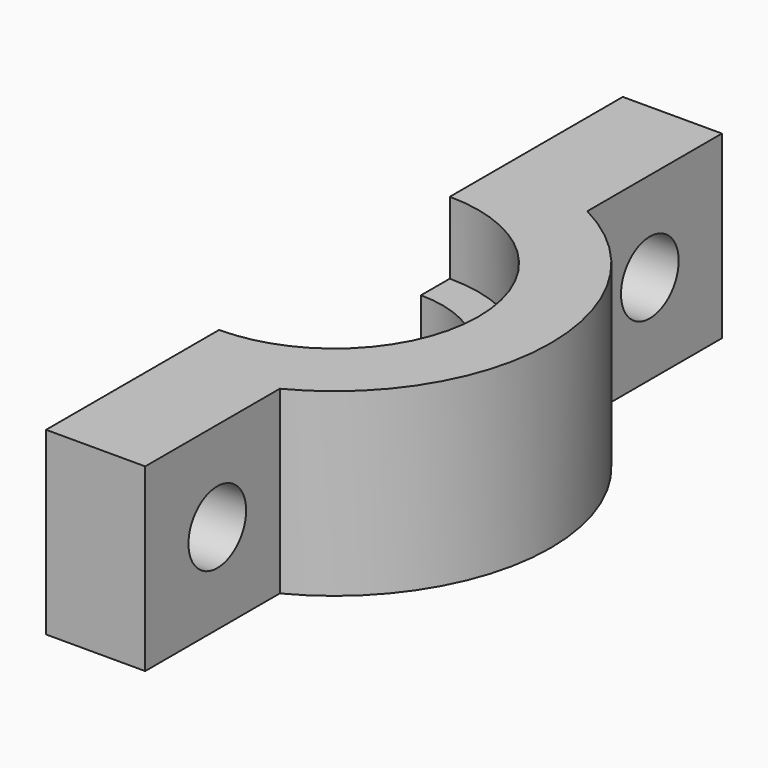
from build123d import *

# Parameters (mm, degrees)
F1_DEPTH = 10
F3_DEPTH = 4
F4_W     = 5.5
F4_H     = 11.188021542
F4_H_2   = 22.7246312633
F4_H_3   = 10.0103956625
F5_DEPTH = 25
F6_DEPTH = 4
F8_D     = 4
F8_DEPTH = 9
F8_TIP   = 1.2017212381


# Not quite as in the source:
# - a feature names something its author has since deleted; it is built from what else it names


with BuildPart() as f1:
    # F0 (on Top) → F1 (new body)
    with BuildSketch(Plane.XY):
        Polygon((60, 11.5470053838), (40, 46.1880215352), (-40, 46.1880215352), (-60, 11.5470053838), (-20, -57.735026919), (20, -57.735026919), align=None)
    extrude(amount=F1_DEPTH)

    # F2 (on face) → F3 (cut)
    with BuildSketch(Plane.XY.offset(10)):
        Polygon((-42.8867513499, 31.188021542), (-48.4529946241, 21.5470053838), (-5.5662432742, -52.7350269258), (5.5662432742, -52.7350269258), (48.4529946241, 21.5470053838), (42.8867513499, 31.188021542), align=None)
    extrude(amount=-F3_DEPTH, mode=Mode.SUBTRACT)

    # F4 (on face) + F1_face (on face) → F5 (cut)
    with BuildSketch(Plane.XY.offset(6)):
        with BuildLine():
            ThreePointArc((-5.5, -10.6653645039), (-12, 0), (-5.5, 10.6653645039))
            Line((-5.5, 10.6653645039), (-5.5, 20))
            Line((-5.5, 20), (-5.5, 31.188021542))
            Line((-5.5, 31.188021542), (-42.8867513499, 31.188021542))
            Line((-42.8867513499, 31.188021542), (-48.4529946241, 21.5470053838))
            Line((-48.4529946241, 21.5470053838), (-11.3457479046, -42.7246312633))
            Line((-11.3457479046, -42.7246312633), (-5.5, -42.7246312633))
            Line((-5.5, -42.7246312633), (-5.5, -20))
            Line((-5.5, -20), (-5.5, -10.6653645039))
        make_face()
        with Locations((2.75, 25.594010771)):
            Rectangle(F4_W, F4_H)
        with Locations((-2.75, 25.594010771)):
            Rectangle(F4_W, F4_H)
        with BuildLine():
            ThreePointArc((-5.5, 10.6653645039), (-2.8298079399, 11.6615688063), (0, 12))
            Line((0, 12), (0, 20))
            Line((0, 20), (-5.5, 20))
            Line((-5.5, 20), (-5.5, 10.6653645039))
        make_face()
        with BuildLine():
            ThreePointArc((-5.5, 5.8094750193), (-2.9600844452, 7.4322204002), (0, 8))
            Line((0, 8), (0, 12))
            ThreePointArc((0, 12), (-2.8298079399, 11.6615688063), (-5.5, 10.6653645039))
            Line((-5.5, 10.6653645039), (-5.5, 5.8094750193))
        make_face()
        with BuildLine():
            ThreePointArc((-5.5, 2.3979157617), (-3.2872865277, 5.0193373352), (0, 6))
            Line((0, 6), (0, 8))
            ThreePointArc((0, 8), (-2.9600844452, 7.4322204002), (-5.5, 5.8094750193))
            Line((-5.5, 5.8094750193), (-5.5, 2.3979157617))
        make_face()
        with BuildLine():
            Line((5.5, -2.3979157617), (5.5, 2.3979157617))
            ThreePointArc((5.5, 2.3979157617), (3.2872865277, 5.0193373352), (0, 6))
            ThreePointArc((0, 6), (-3.2872865277, 5.0193373352), (-5.5, 2.3979157617))
            Line((-5.5, 2.3979157617), (-5.5, -2.3979157617))
            ThreePointArc((-5.5, -2.3979157617), (-3.2872865277, -5.0193373352), (0, -6))
            ThreePointArc((0, -6), (3.2872865277, -5.0193373352), (5.5, -2.3979157617))
        make_face()
        with BuildLine():
            ThreePointArc((-5.5, -2.3979157617), (-6, 0), (-5.5, 2.3979157617))
            Line((-5.5, 2.3979157617), (-5.5, 5.8094750193))
            ThreePointArc((-5.5, 5.8094750193), (-8, 0), (-5.5, -5.8094750193))
            Line((-5.5, -5.8094750193), (-5.5, -2.3979157617))
        make_face()
        with BuildLine():
            ThreePointArc((-5.5, -5.8094750193), (-8, 0), (-5.5, 5.8094750193))
            Line((-5.5, 5.8094750193), (-5.5, 10.6653645039))
            ThreePointArc((-5.5, 10.6653645039), (-12, 0), (-5.5, -10.6653645039))
            Line((-5.5, -10.6653645039), (-5.5, -5.8094750193))
        make_face()
        with BuildLine():
            Line((-5.5, -2.3979157617), (-5.5, 2.3979157617))
            ThreePointArc((-5.5, 2.3979157617), (-6, 0), (-5.5, -2.3979157617))
        make_face()
        with BuildLine():
            Line((0, -8), (0, -6))
            ThreePointArc((0, -6), (-3.2872865277, -5.0193373352), (-5.5, -2.3979157617))
            Line((-5.5, -2.3979157617), (-5.5, -5.8094750193))
            ThreePointArc((-5.5, -5.8094750193), (-2.9600844452, -7.4322204002), (0, -8))
        make_face()
        with BuildLine():
            Line((0, -12), (0, -8))
            ThreePointArc((0, -8), (-2.9600844452, -7.4322204002), (-5.5, -5.8094750193))
            Line((-5.5, -5.8094750193), (-5.5, -10.6653645039))
            ThreePointArc((-5.5, -10.6653645039), (-2.8298079399, -11.6615688063), (0, -12))
        make_face()
        with BuildLine():
            Line((0, -20), (0, -12))
            ThreePointArc((0, -12), (-2.8298079399, -11.6615688063), (-5.5, -10.6653645039))
            Line((-5.5, -10.6653645039), (-5.5, -20))
            Line((-5.5, -20), (0, -20))
        make_face()
        with Locations((-2.75, -31.3623156317)):
            Rectangle(F4_W, F4_H_2)
        with Locations((2.75, -31.3623156317)):
            Rectangle(F4_W, F4_H_2)
        with BuildLine():
            Line((5.5, 20), (5.5, 10.6653645039))
            ThreePointArc((5.5, 10.6653645039), (10.246950766, 6.2449979984), (12, 0))
            ThreePointArc((12, 0), (10.246950766, -6.2449979984), (5.5, -10.6653645039))
            Line((5.5, -10.6653645039), (5.5, -20))
            Line((5.5, -20), (5.5, -42.7246312633))
            Line((5.5, -42.7246312633), (11.3457479046, -42.7246312633))
            Line((11.3457479046, -42.7246312633), (48.4529946241, 21.5470053838))
            Line((48.4529946241, 21.5470053838), (42.8867513499, 31.188021542))
            Line((42.8867513499, 31.188021542), (5.5, 31.188021542))
            Line((5.5, 31.188021542), (5.5, 20))
        make_face()
        Polygon((11.3457479046, -42.7246312633), (5.5, -42.7246312633), (5.5, -52.7350269258), (5.5662432742, -52.7350269258), align=None)
        with Locations((2.75, -47.7298290946)):
            Rectangle(F4_W, F4_H_3)
        with Locations((-2.75, -47.7298290946)):
            Rectangle(F4_W, F4_H_3)
        Polygon((-5.5, -52.7350269258), (-5.5, -42.7246312633), (-11.3457479046, -42.7246312633), (-5.5662432742, -52.7350269258), align=None)
        with BuildLine():
            ThreePointArc((5.5, -2.3979157617), (5.8736700622, -1.2247448714), (6, 0))
            ThreePointArc((6, 0), (5.8736700622, 1.2247448714), (5.5, 2.3979157617))
            Line((5.5, 2.3979157617), (5.5, -2.3979157617))
        make_face()
    with BuildSketch(Plane.XY.offset(10)):
        Polygon((60, 11.5470053838), (40, 46.1880215352), (-40, 46.1880215352), (-60, 11.5470053838), (-20, -57.735026919), (20, -57.735026919), align=None)
        Polygon((-48.4529946241, 21.5470053838), (-42.8867513499, 31.188021542), (42.8867513499, 31.188021542), (48.4529946241, 21.5470053838), (5.5662432742, -52.7350269258), (-5.5662432742, -52.7350269258), align=None, mode=Mode.SUBTRACT)
    extrude(amount=-F5_DEPTH, mode=Mode.SUBTRACT)

    # F4 (on face) → F6 (join)
    with BuildSketch(Plane.XY.offset(6)):
        with BuildLine():
            ThreePointArc((0, 12), (2.8298079399, 11.6615688063), (5.5, 10.6653645039))
            Line((5.5, 10.6653645039), (5.5, 20))
            Line((5.5, 20), (0, 20))
            Line((0, 20), (0, 12))
        make_face()
        with BuildLine():
            ThreePointArc((0, 8), (2.9600844452, 7.4322204002), (5.5, 5.8094750193))
            Line((5.5, 5.8094750193), (5.5, 10.6653645039))
            ThreePointArc((5.5, 10.6653645039), (2.8298079399, 11.6615688063), (0, 12))
            Line((0, 12), (0, 8))
        make_face()
        with BuildLine():
            Line((5.5, 10.6653645039), (5.5, 5.8094750193))
            ThreePointArc((5.5, 5.8094750193), (7.3484692283, 3.1622776602), (8, 0))
            ThreePointArc((8, 0), (7.3484692283, -3.1622776602), (5.5, -5.8094750193))
            Line((5.5, -5.8094750193), (5.5, -10.6653645039))
            ThreePointArc((5.5, -10.6653645039), (10.246950766, -6.2449979984), (12, 0))
            ThreePointArc((12, 0), (10.246950766, 6.2449979984), (5.5, 10.6653645039))
        make_face()
        with BuildLine():
            Line((5.5, -10.6653645039), (5.5, -5.8094750193))
            ThreePointArc((5.5, -5.8094750193), (2.9600844452, -7.4322204002), (0, -8))
            Line((0, -8), (0, -12))
            ThreePointArc((0, -12), (2.8298079399, -11.6615688063), (5.5, -10.6653645039))
        make_face()
        with BuildLine():
            Line((5.5, -20), (5.5, -10.6653645039))
            ThreePointArc((5.5, -10.6653645039), (2.8298079399, -11.6615688063), (0, -12))
            Line((0, -12), (0, -20))
            Line((0, -20), (5.5, -20))
        make_face()
    extrude(amount=F6_DEPTH)

    # F8
    with Locations(Plane(origin=(0, 0, 0), x_dir=(0, -1, 0), z_dir=(-1, 0, 0))):
        with Locations((15, 5), (-15, 5)):
            Hole(F8_D / 2, depth=F8_DEPTH)
            with Locations((0, 0, -(F8_DEPTH + F8_TIP / 2))):  # 118° drill point
                Cone(0, F8_D / 2, F8_TIP, mode=Mode.SUBTRACT)


solid = f1.part
